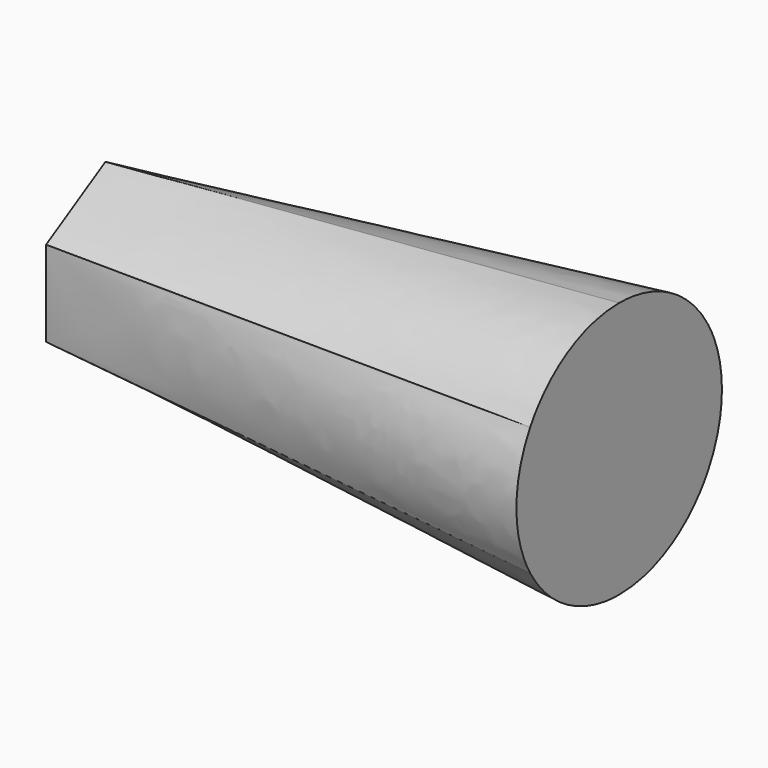
from build123d import *


# Not quite as in the source:
# - the arcs of a loft's sections are written as splines that run evenly, so that the points pair up as in the source's solid


with BuildPart() as f3:
    # F0 (on Right) → F3 section 0
    with BuildSketch(Plane.YZ):
        with BuildLine():
            add(Edge.make_bspline(
                [(64.9519052838, 37.5), (62.7702437188, 41.2787486755), (60.2580232789, 44.8665712892), (54.6486431889, 51.5515701637), (51.5515701637, 54.6486431889), (44.8665712892, 60.2580232789), (41.2787486755, 62.7702437188), (33.7212513245, 67.1335668488), (29.7516932968, 68.9846021566), (21.5513282021, 71.9692909612), (17.3206477723, 73.1028983658), (8.7265788777, 74.618264586), (4.36332313, 75), (0, 75)],
                knots=[0, 0, 0, 0, 0.1666666667, 0.1666666667, 0.3333333333, 0.3333333333, 0.5, 0.5, 0.6666666667, 0.6666666667, 0.8333333333, 0.8333333333, 1, 1, 1, 1], degree=3))
            add(Edge.make_bspline(
                [(0, 75), (-4.36332313, 75), (-8.7265788777, 74.618264586), (-17.3206477723, 73.1028983658), (-21.5513282021, 71.9692909612), (-29.7516932968, 68.9846021566), (-33.7212513245, 67.1335668488), (-41.2787486755, 62.7702437188), (-44.8665712892, 60.2580232789), (-51.5515701637, 54.6486431889), (-54.6486431889, 51.5515701637), (-60.2580232789, 44.8665712892), (-62.7702437188, 41.2787486755), (-64.9519052838, 37.5)],
                knots=[0, 0, 0, 0, 0.1666666667, 0.1666666667, 0.3333333333, 0.3333333333, 0.5, 0.5, 0.6666666667, 0.6666666667, 0.8333333333, 0.8333333333, 1, 1, 1, 1], degree=3))
            add(Edge.make_bspline(
                [(-64.9519052838, 37.5), (-67.1335668488, 33.7212513245), (-68.9846021566, 29.7516932968), (-71.9692909612, 21.5513282021), (-73.1028983658, 17.3206477723), (-74.618264586, 8.7265788777), (-75, 4.36332313), (-75, -4.36332313), (-74.618264586, -8.7265788777), (-73.1028983658, -17.3206477723), (-71.9692909612, -21.5513282021), (-68.9846021566, -29.7516932968), (-67.1335668488, -33.7212513245), (-64.9519052838, -37.5)],
                knots=[0, 0, 0, 0, 0.1666666667, 0.1666666667, 0.3333333333, 0.3333333333, 0.5, 0.5, 0.6666666667, 0.6666666667, 0.8333333333, 0.8333333333, 1, 1, 1, 1], degree=3))
            add(Edge.make_bspline(
                [(-64.9519052838, -37.5), (-62.7702437188, -41.2787486755), (-60.2580232789, -44.8665712892), (-54.6486431889, -51.5515701637), (-51.5515701637, -54.6486431889), (-44.8665712892, -60.2580232789), (-41.2787486755, -62.7702437188), (-33.7212513245, -67.1335668488), (-29.7516932968, -68.9846021566), (-21.5513282021, -71.9692909612), (-17.3206477723, -73.1028983658), (-8.7265788777, -74.618264586), (-4.36332313, -75), (0, -75)],
                knots=[0, 0, 0, 0, 0.1666666667, 0.1666666667, 0.3333333333, 0.3333333333, 0.5, 0.5, 0.6666666667, 0.6666666667, 0.8333333333, 0.8333333333, 1, 1, 1, 1], degree=3))
            add(Edge.make_bspline(
                [(0, -75), (4.36332313, -75), (8.7265788777, -74.618264586), (17.3206477723, -73.1028983658), (21.5513282021, -71.9692909612), (29.7516932968, -68.9846021566), (33.7212513245, -67.1335668488), (41.2787486755, -62.7702437188), (44.8665712892, -60.2580232789), (51.5515701637, -54.6486431889), (54.6486431889, -51.5515701637), (60.2580232789, -44.8665712892), (62.7702437188, -41.2787486755), (64.9519052838, -37.5)],
                knots=[0, 0, 0, 0, 0.1666666667, 0.1666666667, 0.3333333333, 0.3333333333, 0.5, 0.5, 0.6666666667, 0.6666666667, 0.8333333333, 0.8333333333, 1, 1, 1, 1], degree=3))
            add(Edge.make_bspline(
                [(64.9519052838, -37.5), (67.1335668488, -33.7212513245), (68.9846021566, -29.7516932968), (71.9692909612, -21.5513282021), (73.1028983658, -17.3206477723), (74.618264586, -8.7265788777), (75, -4.36332313), (75, 4.36332313), (74.618264586, 8.7265788777), (73.1028983658, 17.3206477723), (71.9692909612, 21.5513282021), (68.9846021566, 29.7516932968), (67.1335668488, 33.7212513245), (64.9519052838, 37.5)],
                knots=[0, 0, 0, 0, 0.1666666667, 0.1666666667, 0.3333333333, 0.3333333333, 0.5, 0.5, 0.6666666667, 0.6666666667, 0.8333333333, 0.8333333333, 1, 1, 1, 1], degree=3))
        make_face()
    # F2 (on offset) → F3 section 1
    with BuildSketch(Plane.YZ.offset(-300)):
        Polygon((43.3012701892, 25), (0, 50), (-43.3012701892, 25), (-43.3012701892, -25), (0, -50), (43.3012701892, -25), align=None)
    loft(ruled=True)


solid = f3.part
